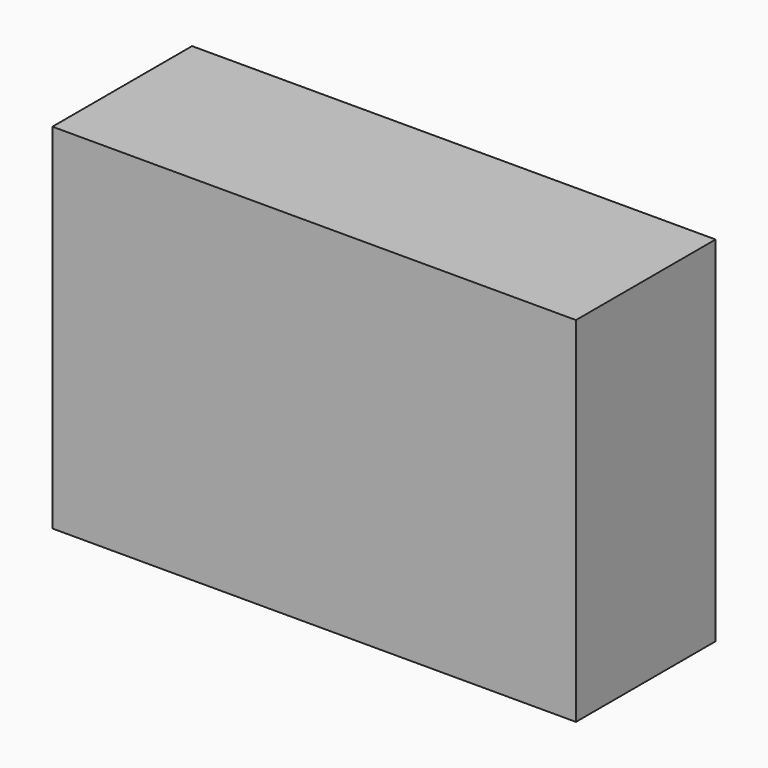
from build123d import *

# Parameters (mm, degrees)
F0_W     = 76.2000083923
F0_H     = 51.4927282929
F3_DEPTH = 25.4


# Not quite as in the source:
# - the program builds the solid bodies; features that only make, move or delete a surface that nothing else refers to are left out


with BuildPart() as f3:
    # F0 (on Front) → F3 (new body)
    with BuildSketch(Plane.XZ):
        Rectangle(F0_W, F0_H)
    extrude(amount=-F3_DEPTH)


solid = f3.part
